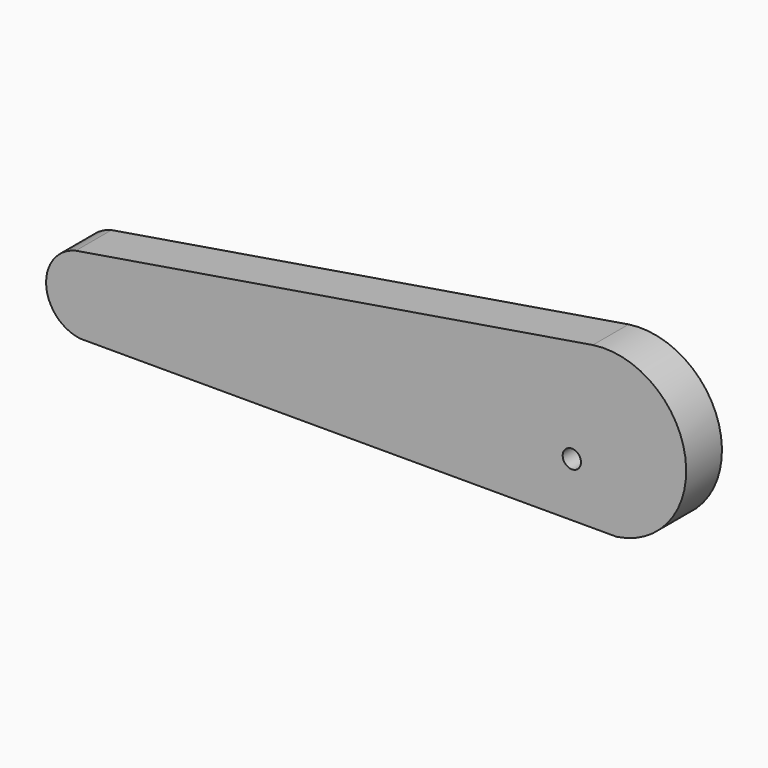
from build123d import *

# Parameters (mm, degrees)
F1_DEPTH = 8.73125
F2_R     = 1.7859375
F3_DEPTH = 8.73125


# Not quite as in the source:
# - a length typed as a fraction of an inch, garbled in the dataset ("3 / 203.2 mm" for 3/8 in), is restored


with BuildPart() as f1:
    # F0 (on Front) → F1 (new body)
    with BuildSketch(Plane.XZ):
        with BuildLine():
            Line((16.3863981424, 24.04380231), (-84.6225991332, 7.4210920542))
            ThreePointArc((-84.6225991332, 7.4210920542), (-90.4179458573, -0.3797760525), (-83.7262291187, -7.42679769))
            Line((-83.7262291187, -7.42679769), (21.0487708813, -7.42679769))
            ThreePointArc((21.0487708813, -7.42679769), (34.4528845118, 10.6396886794), (16.3863981424, 24.04380231))
        make_face()
    extrude(amount=F1_DEPTH)

    # F2 (on face) → F3 (cut, through all)
    with BuildSketch(Plane.XZ.offset(8.73125)):
        with Locations((12.2811356559, 3.1172726303)):
            Circle(F2_R)
    extrude(amount=-F3_DEPTH, mode=Mode.SUBTRACT)


solid = f1.part
